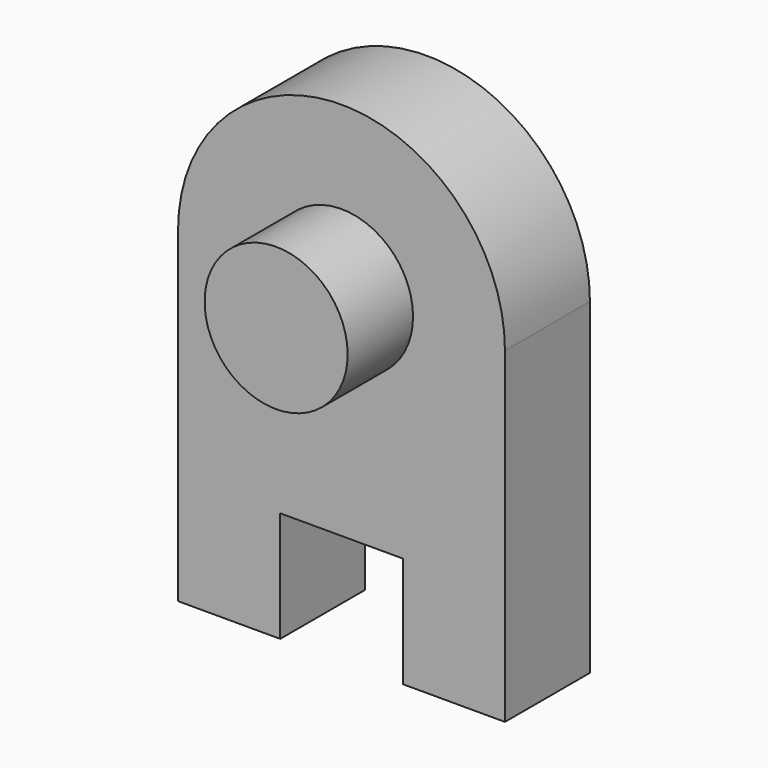
from build123d import *

# Parameters (mm, degrees)
F0_W     = 762
F0_H     = 635
F1_DEPTH = 635
F2_DEPTH = 25.4
F3_W     = 762
F3_H     = 1322.5318927765
F4_DEPTH = 660.401
F5_R     = 444.5
F6_DEPTH = 508


with BuildPart() as f1:
    # F0 (on Front) → F1 (new body)
    with BuildSketch(Plane.XZ):
        with BuildLine():
            ThreePointArc((-1016, 1016), (0, 0), (1016, 1016))
            Line((1016, 1016), (-1016, 1016))
        make_face()
        with Locations((0, -1333.5)):
            Rectangle(F0_W, F0_H)
        with BuildLine():
            Line((381, -1016), (1016, -1016))
            Line((1016, -1016), (1016, 1016))
            ThreePointArc((1016, 1016), (0, 0), (-1016, 1016))
            Line((-1016, 1016), (-1016, -1016))
            Line((-1016, -1016), (-381, -1016))
            Line((-381, -1016), (-381, -381))
            Line((-381, -381), (381, -381))
            Line((381, -381), (381, -1016))
        make_face()
        with Locations((0, -698.5)):
            Rectangle(F0_W, F0_H)
        with BuildLine():
            Line((-1016, 1016), (1016, 1016))
            ThreePointArc((1016, 1016), (0, 2032), (-1016, 1016))
        make_face()
    extrude(amount=F1_DEPTH)

    # F2 (add): a face of the model
    f2_faces = [f1.faces().sort_by_distance(p)[0] for p in [
        (0, -635, 272.8986892682),
    ]]
    extrude(f2_faces, amount=F2_DEPTH)

    # F3 (on face) → F4 (cut, through all)
    with BuildSketch(Plane.XZ.offset(660.4)):
        with Locations((0, -989.7340536118)):
            Rectangle(F3_W, F3_H)
    extrude(amount=-F4_DEPTH, mode=Mode.SUBTRACT)

    # F5 (on face) → F6 (join)
    with BuildSketch(Plane.XZ.offset(660.4)):
        with Locations((0, 1016)):
            Circle(F5_R)
    extrude(amount=F6_DEPTH)


solid = f1.part
